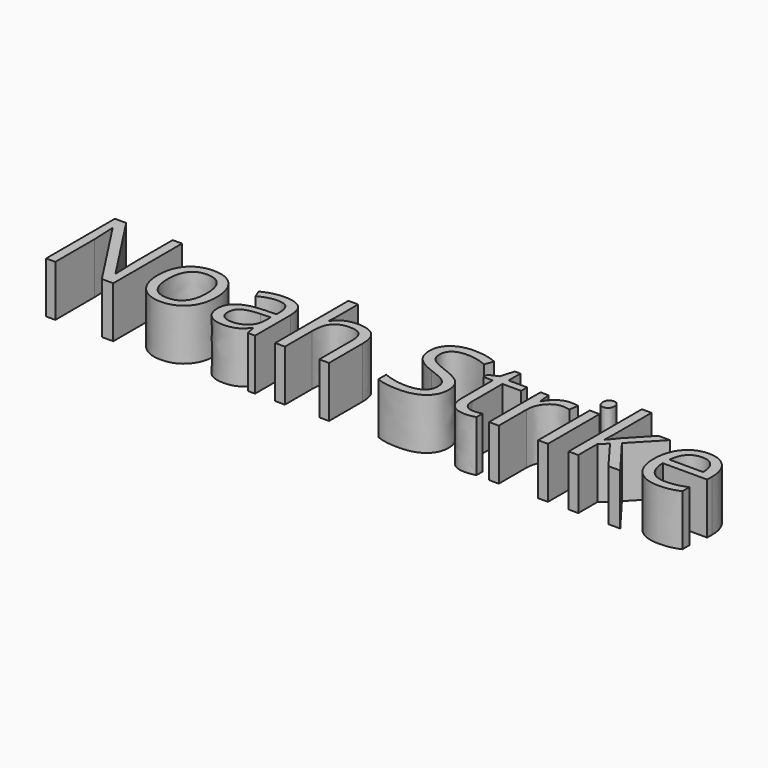
from build123d import *

# Parameters (mm, degrees)
F0_TEXT_SIZE = 5.9871673462
F1_DEPTH     = 2.54


# Not quite as in the source:
# - Text() gives the source's letters only with a copy of the font that has no kerning and outlines rounded to 1/6400 em; it was checked with that copy


with BuildPart() as f1:
    # F0 (on Top) → F1 (new body)
    with BuildSketch(Plane.XY):
        with Locations((0, -4.3107604893)):
            Text('Noah Strike', F0_TEXT_SIZE, font='Open Sans', text_align=(TextAlign.LEFT, TextAlign.BOTTOM))
    extrude(amount=F1_DEPTH)


solid = f1.part
